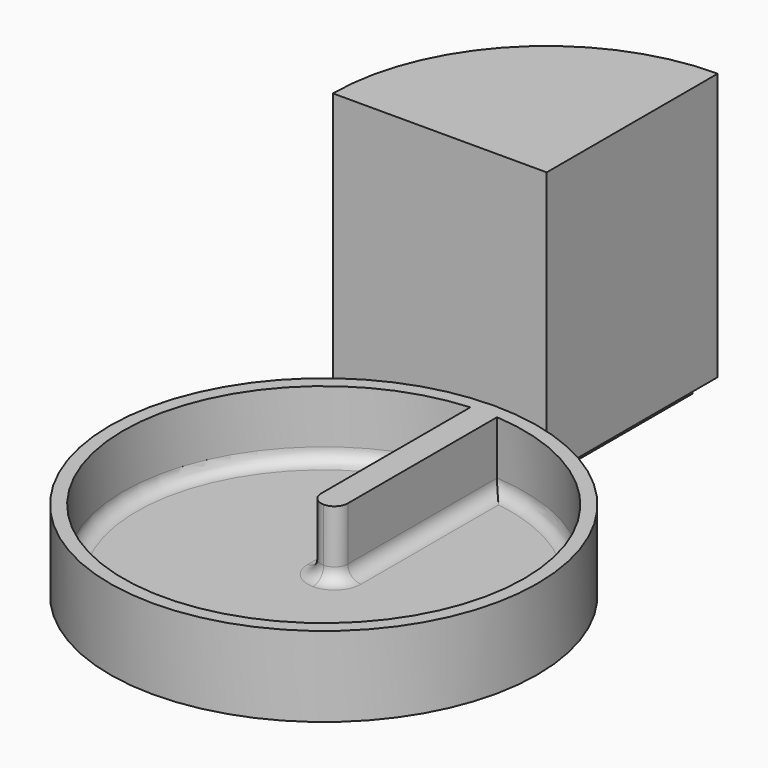
from build123d import *

# Parameters (mm, degrees)
F0_R      = 50.8
F1_DEPTH  = 19.05
F2_T      = -3.175
F4_DEPTH  = 15.875
F5_R      = 3.17499
F7_DEPTH  = 63.5
F8_T      = -3.175
F10_DEPTH = 3.175
F11_R     = 3.175
F12_DEPTH = 25.4


# Not quite as in the source:
# - a fillet or chamfer is up to 0.001 mm smaller than in the source, because OpenCascade refuses the exact size


with BuildPart() as f1:
    # F0 (on Top) → F1 (new body)
    with BuildSketch(Plane.XY):
        Circle(F0_R)
    extrude(amount=F1_DEPTH)

    # F2
    f2_openings = [f1.faces().sort_by_distance(p)[0] for p in [
        (0, 0, 19.05),
    ]]
    offset(amount=F2_T, openings=f2_openings)

    # F3 (on face) → F4 (join, through all)
    with BuildSketch(Plane.XY.offset(3.175)):
        with BuildLine():
            Line((-3.175, 0), (0, 0))
            Line((0, 0), (3.175, 0))
            Line((3.175, 0), (3.175, 47.519048812))
            ThreePointArc((3.175, 47.519048812), (0, 47.625), (-3.175, 47.519048812))
            Line((-3.175, 47.519048812), (-3.175, 0))
        make_face()
    extrude(amount=F4_DEPTH)

    # F5 (radius 3.175 in the source; OpenCascade refuses exactly that, so slightly less here)
    f5_edges = [f1.edges().sort_by_distance(p)[0] for p in [
        (34.780382, 32.534069, 3.175),
        (-32.534069, -34.780382, 3.175),
        (-3.175, 23.759524, 3.175),
        (0, 0, 3.175),
        (3.175, 23.759524, 3.175),
        (3.175, 0, 11.1125),
        (-3.175, 0, 11.1125),
    ]]
    fillet(f5_edges, radius=F5_R)


with BuildPart() as f7:
    # F6 (on Top) → F7 (new body)
    with BuildSketch(Plane.XY):
        with BuildLine():
            Line((-48.5592149198, 63.44383955), (2.2407850802, 63.44383955))
            Line((2.2407850802, 63.44383955), (2.2407850802, 114.24383955))
            ThreePointArc((2.2407850802, 114.24383955), (-33.6802394041, 99.3648640343), (-48.5592149198, 63.44383955))
        make_face()
    extrude(amount=F7_DEPTH)

    # F8 (hollow: no face is removed)
    offset(amount=F8_T, mode=Mode.SUBTRACT)

    # F9 (on face) → F10 (join)
    with BuildSketch(Plane(origin=(0, 0, 0), x_dir=(1, 0, 0), z_dir=(0, 0, -1))):
        with BuildLine():
            Line((-1.0612149198, -110.8269251397), (-1.0612149198, -66.74583955))
            Line((-1.0612149198, -66.74583955), (-45.1423005095, -66.74583955))
            ThreePointArc((-45.1423005095, -66.74583955), (-31.3453728126, -97.0299974428), (-1.0612149198, -110.8269251397))
        make_face()
    extrude(amount=F10_DEPTH)

    # F11 (on face) → F12 (cut)
    with BuildSketch(Plane(origin=(0, 0, -3.175), x_dir=(1, 0, 0), z_dir=(0, 0, -1))):
        with Locations((-10.4592149198, -76.14383955)):
            Circle(F11_R)
    extrude(amount=-F12_DEPTH, mode=Mode.SUBTRACT)


solid = Compound([f1.part, f7.part])
